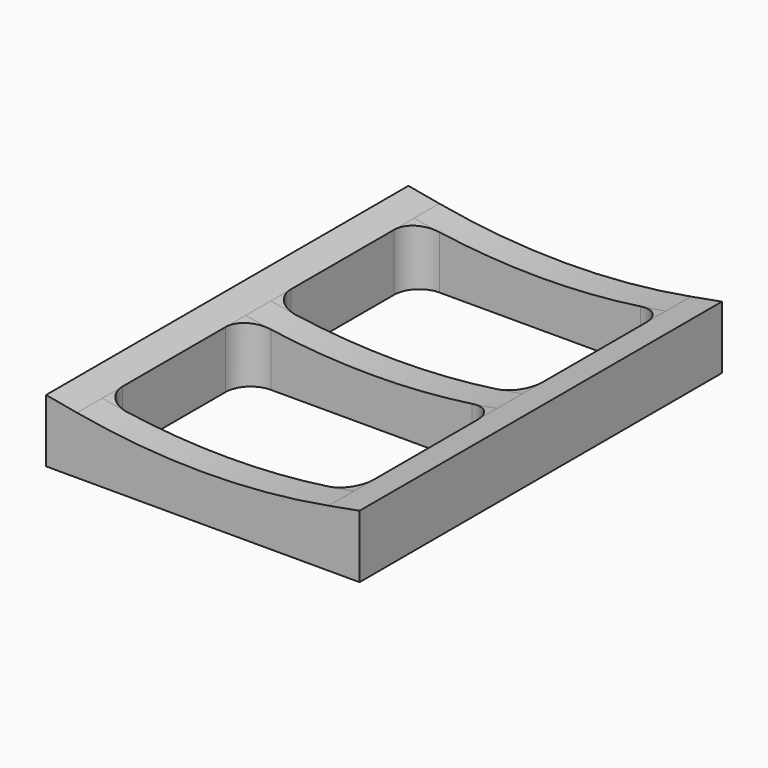
from build123d import *

# Parameters (mm, degrees)
F1_DEPTH     = 45.72
F2_DEPTH     = 39.37
F3_DEPTH     = 3.175
F4_T4_DEPTH  = 24.2661839103
F4_S5_R      = 142.2541111111
F4_T6_DEPTH  = 14
F4_T10_DEPTH = 24.2661839103
F4_S11_R     = 142.2541111111
F4_T12_DEPTH = 14
F4_T16_DEPTH = 24.2661839103
F4_S17_R     = 142.2541111111
F4_T18_DEPTH = 14
F4_T22_DEPTH = 24.2661839103
F4_S23_R     = 142.2541111111
F4_T24_DEPTH = 14
F4_T28_DEPTH = 24.2661839103
F4_S29_R     = 142.2541111111
F4_T30_DEPTH = 14
F4_T34_DEPTH = 24.2661839103
F4_S35_R     = 142.2541111111
F4_T36_DEPTH = 14
F4_T40_DEPTH = 24.2661839103
F4_S41_R     = 142.2541111111
F4_T42_DEPTH = 14
F4_T46_DEPTH = 24.2661839103
F4_S47_R     = 142.2541111111
F4_T48_DEPTH = 14


# Not quite as in the source:
# - a fillet or chamfer that OpenCascade refuses, or shapes differently, is made with other operations: its cross-section is extruded or revolved along the edge and cut away or added


with BuildPart() as f1:
    # F0 (on Front) → F1 (new body, symmetric)
    with BuildSketch(Plane.XZ):
        with BuildLine():
            ThreePointArc((25.4, 11.5661839103), (12.7513312638, 9.8528365344), (0, 9.2801839103))
            ThreePointArc((0, 9.2801839103), (-12.7513312638, 9.8528365344), (-25.4, 11.5661839103))
            Line((-25.4, 11.5661839103), (-25.4, 0))
            Line((-25.4, 0), (25.4, 0))
            Line((25.4, 0), (25.4, 11.5661839103))
        make_face()
        Polygon((-25.4, 0), (-25.4, 11.5661839103), (-31.6479565519, 12.7), (-31.6479565519, 0), align=None)
        Polygon((31.6479565519, 12.7), (25.4, 11.5661839103), (25.4, 0), (31.6479565519, 0), align=None)
    extrude(amount=F1_DEPTH, both=True)

    # F0 (on Front) → F2 (cut, symmetric)
    with BuildSketch(Plane.XZ):
        with BuildLine():
            ThreePointArc((25.4, 11.5661839103), (12.7513312638, 9.8528365344), (0, 9.2801839103))
            ThreePointArc((0, 9.2801839103), (-12.7513312638, 9.8528365344), (-25.4, 11.5661839103))
            Line((-25.4, 11.5661839103), (-25.4, 0))
            Line((-25.4, 0), (25.4, 0))
            Line((25.4, 0), (25.4, 11.5661839103))
        make_face()
    extrude(amount=F2_DEPTH, both=True, mode=Mode.SUBTRACT)

    # F0 (on Front) → F3 (join, symmetric)
    with BuildSketch(Plane.XZ):
        with BuildLine():
            ThreePointArc((25.4, 11.5661839103), (12.7513312638, 9.8528365344), (0, 9.2801839103))
            ThreePointArc((0, 9.2801839103), (-12.7513312638, 9.8528365344), (-25.4, 11.5661839103))
            Line((-25.4, 11.5661839103), (-25.4, 0))
            Line((-25.4, 0), (25.4, 0))
            Line((25.4, 0), (25.4, 11.5661839103))
        make_face()
    extrude(amount=F3_DEPTH, both=True)

    # F4: fillet of radius 5.08 on 8 edges, made by hand


with BuildPart() as f4_tool2:
    # F4_s3 → F4_t4 (new body)
    with BuildSketch(Plane.XY.offset(24.2661839103)):
        with BuildLine():
            ThreePointArc((-20.32, 39.37), (-23.9121024484, 37.8821024484), (-25.4, 34.29))
            Line((-25.4, 34.29), (-25.4, 39.37))
            Line((-25.4, 39.37), (-20.32, 39.37))
        make_face()
    extrude(amount=-F4_T4_DEPTH)

    # F4_s5 → F4_t6 (cut, symmetric)
    with BuildSketch(Plane.XZ.offset(-36.8)):
        with Locations((0, 151.5342950214)):
            Circle(F4_S5_R)
    extrude(amount=F4_T6_DEPTH, both=True, mode=Mode.SUBTRACT)


with BuildPart() as f1_1:
    add(f1.part)

    # F4_t1: union F4_tool2
    add(f4_tool2.part)


with BuildPart() as f4_tool8:
    # F4_s9 → F4_t10 (new body)
    with BuildSketch(Plane.XY):
        with BuildLine():
            ThreePointArc((20.32, 39.37), (23.9121024484, 37.8821024484), (25.4, 34.29))
            Line((25.4, 34.29), (25.4, 39.37))
            Line((25.4, 39.37), (20.32, 39.37))
        make_face()
    extrude(amount=F4_T10_DEPTH)

    # F4_s11 → F4_t12 (cut, symmetric)
    with BuildSketch(Plane.XZ.offset(-36.8)):
        with Locations((0, 151.5342950214)):
            Circle(F4_S11_R)
    extrude(amount=F4_T12_DEPTH, both=True, mode=Mode.SUBTRACT)


with BuildPart() as f1_2:
    add(f1_1.part)

    # F4_t7: union F4_tool8
    add(f4_tool8.part)


with BuildPart() as f4_tool14:
    # F4_s15 → F4_t16 (new body)
    with BuildSketch(Plane.XY):
        with BuildLine():
            ThreePointArc((25.4, -8.255), (23.9121024484, -4.6628975516), (20.32, -3.175))
            Line((20.32, -3.175), (25.4, -3.175))
            Line((25.4, -3.175), (25.4, -8.255))
        make_face()
    extrude(amount=F4_T16_DEPTH)

    # F4_s17 → F4_t18 (cut, symmetric)
    with BuildSketch(Plane.XZ.offset(5.7)):
        with Locations((0, 151.5342950214)):
            Circle(F4_S17_R)
    extrude(amount=F4_T18_DEPTH, both=True, mode=Mode.SUBTRACT)


with BuildPart() as f1_3:
    add(f1_2.part)

    # F4_t13: union F4_tool14
    add(f4_tool14.part)


with BuildPart() as f4_tool20:
    # F4_s21 → F4_t22 (new body)
    with BuildSketch(Plane.XY.offset(24.2661839103)):
        with BuildLine():
            ThreePointArc((-25.4, -8.255), (-23.9121024484, -4.6628975516), (-20.32, -3.175))
            Line((-20.32, -3.175), (-25.4, -3.175))
            Line((-25.4, -3.175), (-25.4, -8.255))
        make_face()
    extrude(amount=-F4_T22_DEPTH)

    # F4_s23 → F4_t24 (cut, symmetric)
    with BuildSketch(Plane.XZ.offset(5.7)):
        with Locations((0, 151.5342950214)):
            Circle(F4_S23_R)
    extrude(amount=F4_T24_DEPTH, both=True, mode=Mode.SUBTRACT)


with BuildPart() as f1_4:
    add(f1_3.part)

    # F4_t19: union F4_tool20
    add(f4_tool20.part)


with BuildPart() as f4_tool26:
    # F4_s27 → F4_t28 (new body)
    with BuildSketch(Plane.XY):
        with BuildLine():
            ThreePointArc((25.4, 8.255), (23.9121024484, 4.6628975516), (20.32, 3.175))
            Line((20.32, 3.175), (25.4, 3.175))
            Line((25.4, 3.175), (25.4, 8.255))
        make_face()
    extrude(amount=F4_T28_DEPTH)

    # F4_s29 → F4_t30 (cut, symmetric)
    with BuildSketch(Plane.XZ.offset(-5.7)):
        with Locations((0, 151.5342950214)):
            Circle(F4_S29_R)
    extrude(amount=F4_T30_DEPTH, both=True, mode=Mode.SUBTRACT)


with BuildPart() as f1_5:
    add(f1_4.part)

    # F4_t25: union F4_tool26
    add(f4_tool26.part)


with BuildPart() as f4_tool32:
    # F4_s33 → F4_t34 (new body)
    with BuildSketch(Plane.XY):
        with BuildLine():
            ThreePointArc((25.4, -34.29), (23.9121024484, -37.8821024484), (20.32, -39.37))
            Line((20.32, -39.37), (25.4, -39.37))
            Line((25.4, -39.37), (25.4, -34.29))
        make_face()
    extrude(amount=F4_T34_DEPTH)

    # F4_s35 → F4_t36 (cut, symmetric)
    with BuildSketch(Plane.XZ.offset(36.8)):
        with Locations((0, 151.5342950214)):
            Circle(F4_S35_R)
    extrude(amount=F4_T36_DEPTH, both=True, mode=Mode.SUBTRACT)


with BuildPart() as f1_6:
    add(f1_5.part)

    # F4_t31: union F4_tool32
    add(f4_tool32.part)


with BuildPart() as f4_tool38:
    # F4_s39 → F4_t40 (new body)
    with BuildSketch(Plane.XY.offset(24.2661839103)):
        with BuildLine():
            ThreePointArc((-25.4, -34.29), (-23.9121024484, -37.8821024484), (-20.32, -39.37))
            Line((-20.32, -39.37), (-25.4, -39.37))
            Line((-25.4, -39.37), (-25.4, -34.29))
        make_face()
    extrude(amount=-F4_T40_DEPTH)

    # F4_s41 → F4_t42 (cut, symmetric)
    with BuildSketch(Plane.XZ.offset(36.8)):
        with Locations((0, 151.5342950214)):
            Circle(F4_S41_R)
    extrude(amount=F4_T42_DEPTH, both=True, mode=Mode.SUBTRACT)


with BuildPart() as f1_7:
    add(f1_6.part)

    # F4_t37: union F4_tool38
    add(f4_tool38.part)


with BuildPart() as f4_tool44:
    # F4_s45 → F4_t46 (new body)
    with BuildSketch(Plane.XY.offset(24.2661839103)):
        with BuildLine():
            ThreePointArc((-25.4, 8.255), (-23.9121024484, 4.6628975516), (-20.32, 3.175))
            Line((-20.32, 3.175), (-25.4, 3.175))
            Line((-25.4, 3.175), (-25.4, 8.255))
        make_face()
    extrude(amount=-F4_T46_DEPTH)

    # F4_s47 → F4_t48 (cut, symmetric)
    with BuildSketch(Plane.XZ.offset(-5.7)):
        with Locations((0, 151.5342950214)):
            Circle(F4_S47_R)
    extrude(amount=F4_T48_DEPTH, both=True, mode=Mode.SUBTRACT)


with BuildPart() as f1_8:
    add(f1_7.part)

    # F4_t43: union F4_tool44
    add(f4_tool44.part)


solid = f1_8.part
